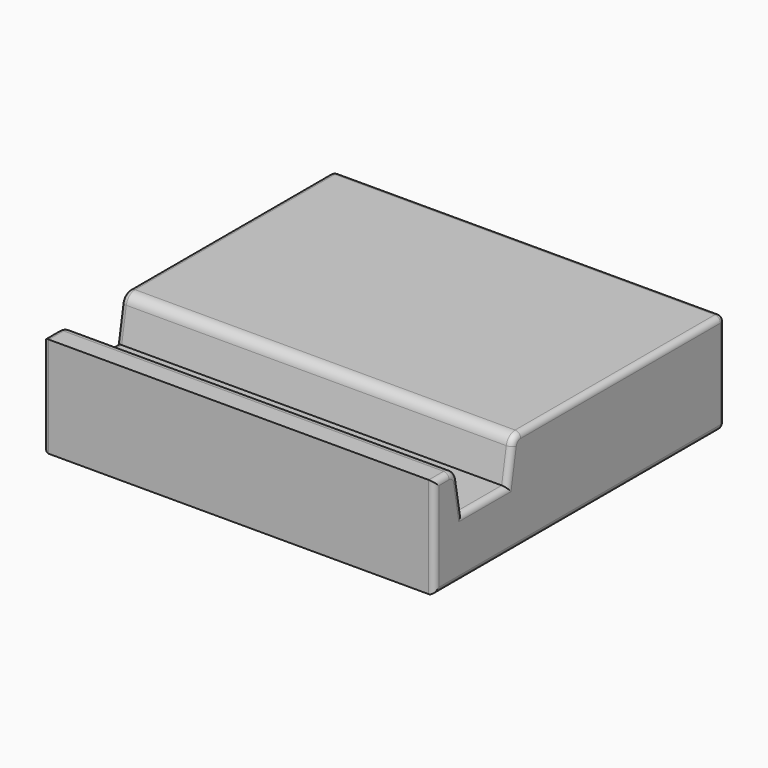
from build123d import *

# Parameters (mm, degrees)
F0_W          = 65
F0_H          = 18
F1_DEPTH      = 35
F3_DEPTH      = 70.001
F4_R          = 2
F5_R          = 1
F6_W          = 7
F6_H          = 3
F7_DEPTH      = 7.5
F8_W          = 58
F8_H          = 50
F9_DEPTH      = 7
F10_T1_DEPTH  = 50
F10_T3_DEPTH  = 58
F10_T8_DEPTH  = 65.7150489639
F10_T13_DEPTH = 58
F10_T18_DEPTH = 65.7150489639


# Not quite as in the source:
# - a fillet or chamfer that OpenCascade refuses, or shapes differently, is made with other operations: its cross-section is extruded or revolved along the edge and cut away or added


with BuildPart() as f1:
    # F0 (on Right) → F1 (new body, symmetric)
    with BuildSketch(Plane.YZ):
        Rectangle(F0_W, F0_H)
    extrude(amount=F1_DEPTH, both=True)

    # F2 (on face) → F3 (cut, through all)
    with BuildSketch(Plane.YZ.offset(35)):
        Polygon((-14.8550952894, 9), (-27.5, 9), (-26.1775476447, 1.5), (-16.1775476447, 1.5), align=None)
        Polygon((-21.5490479022, 13.5265095159), (-32.5, 9), (-27.5, 9), (-14.8550952894, 9), align=None)
    extrude(amount=-F3_DEPTH, mode=Mode.SUBTRACT)

    # F4
    f4_edges = [f1.edges().sort_by_distance(p)[0] for p in [
        (0, -14.855095, 9),
        (0, -27.5, 9),
    ]]
    fillet(f4_edges, radius=F4_R)

    # F5
    f5_edges = [f1.edges().sort_by_distance(p)[0] for p in [
        (35, 9.661552, 9),
        (35, -30.8391, 9),
        (35, -27.892624, 8.532089),
        (35, -32.5, 0),
        (35, -26.693066, 4.423648),
        (35, 0, -9),
        (35, -21.177548, 1.5),
        (35, 32.5, 0),
        (35, -15.66203, 4.423648),
        (35, -14.462471, 8.532089),
        (-35, 32.5, 0),
        (0, 32.5, 9),
        (0, 32.5, -9),
        (-35, -30.8391, 9),
        (-35, -27.892624, 8.532089),
        (-35, -32.5, 0),
        (-35, -26.693066, 4.423648),
        (-35, 0, -9),
        (-35, -21.177548, 1.5),
        (-35, -15.66203, 4.423648),
        (-35, 9.661552, 9),
        (-35, -14.462471, 8.532089),
    ]]
    fillet(f5_edges, radius=F5_R)

    # F6 (on Right) → F7 (cut, symmetric)
    with BuildSketch(Plane.YZ):
        with Locations((-21.1775476447, -1)):
            Rectangle(F6_W, F6_H)
        with Locations((-21.1775476447, 2)):
            Rectangle(F6_W, F6_H)
    extrude(amount=F7_DEPTH, both=True, mode=Mode.SUBTRACT)

    # F8 (on face) → F9 (cut)
    with BuildSketch(Plane(origin=(0, 0, -9), x_dir=(1, 0, 0), z_dir=(0, 0, -1))):
        Rectangle(F8_W, F8_H)
    extrude(amount=-F9_DEPTH, mode=Mode.SUBTRACT)

    # F10: chamfer of 3 on 4 edges, made by hand

    # F10_s2 → F10_t1 (join)
    with BuildSketch(Plane.XZ.offset(-25)):
        Polygon((26, -2), (29, -5), (29, -2), align=None)
        Polygon((-26, -2), (-29, -5), (-29, -2), align=None)
    extrude(amount=F10_T1_DEPTH)

    # F10_s4 → F10_t3 (join)
    with BuildSketch(Plane.YZ.offset(-29)):
        Polygon((22, -2), (25, -5), (25, -2), align=None)
    extrude(amount=F10_T3_DEPTH)


with BuildPart() as f10_tool6:
    # F10_s7 → F10_t8 (new body)
    with BuildSketch(Plane.YZ.offset(29)):
        Polygon((-22, -2), (-25, -5), (-25, -2), align=None)
    extrude(amount=-F10_T8_DEPTH)

    split(bisect_by=Plane.YZ.offset(7.5), keep=Keep.TOP)


with BuildPart() as f1_1:
    add(f1.part)

    # F10_t5: union F10_tool6
    add(f10_tool6.part)


with BuildPart() as f10_tool11:
    # F10_s12 → F10_t13 (new body)
    with BuildSketch(Plane.YZ.offset(29)):
        Polygon((-22, -2), (-25, -5), (-25, -2), align=None)
    extrude(amount=-F10_T13_DEPTH)

    split(bisect_by=Plane.XZ.offset(24.6775476447), keep=Keep.TOP)


with BuildPart() as f1_2:
    add(f1_1.part)

    # F10_t10: union F10_tool11
    add(f10_tool11.part)


with BuildPart() as f10_tool16:
    # F10_s17 → F10_t18 (new body)
    with BuildSketch(Plane.YZ.offset(36.7150489639)):
        Polygon((-22, -2), (-25, -5), (-25, -2), align=None)
    extrude(amount=-F10_T18_DEPTH)

    split(bisect_by=Plane.YZ.offset(-7.5), keep=Keep.BOTTOM)


with BuildPart() as f1_3:
    add(f1_2.part)

    # F10_t15: union F10_tool16
    add(f10_tool16.part)


solid = f1_3.part
